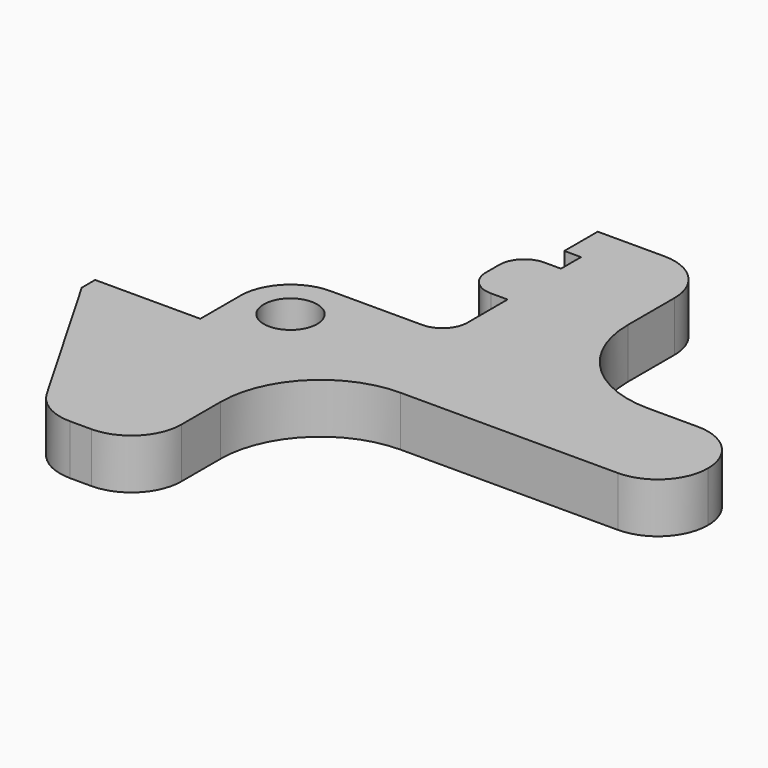
from build123d import *

# Parameters (mm, degrees)
F0_R     = 1.6
F0_W     = 6.3
F0_H     = 1
F0_W_2   = 2.5
F0_H_2   = 4
F1_DEPTH = 3
F2_R     = 2.99999
F3_R     = 6
F4_R     = 1.5


# Not quite as in the source:
# - a fillet or chamfer is up to 0.001 mm smaller than in the source, because OpenCascade refuses the exact size


with BuildPart() as f1:
    # F0 (on Top) → F1 (new body)
    with BuildSketch(Plane.XY):
        with BuildLine():
            ThreePointArc((0, 3), (-2.1213203436, 2.1213203436), (-3, 0))
            Line((-3, 0), (-3, -3))
            Line((-3, -3), (-3, -4))
            Line((-3, -4), (-9.3, -4))
            Line((-9.3, -4), (-3, -14.9119200877))
            Line((-3, -14.9119200877), (3, -14.9119200877))
            Line((3, -14.9119200877), (3, -3))
            Line((3, -3), (25, -3))
            Line((25, -3), (25, 3))
            Line((25, 3), (13, 3))
            Line((13, 3), (7, 3))
            Line((7, 3), (0, 3))
        make_face()
        Circle(F0_R, mode=Mode.SUBTRACT)
        with Locations((-6.15, -3.5)):
            Rectangle(F0_W, F0_H)
        Polygon((7, 7.5), (7, 3), (13, 3), (13, 13), (7, 13), (7, 11.5), align=None)
        with Locations((5.75, 9.5)):
            Rectangle(F0_W_2, F0_H_2)
        Polygon((7, 13), (13, 13), (13, 15.5), (6, 15.5), (6, 13), align=None)
    extrude(amount=F1_DEPTH)

    # F2 (radius 3 in the source; OpenCascade refuses exactly that, so slightly less here)
    f2_edges = [f1.edges().sort_by_distance(p)[0] for p in [
        (-3, -14.91192, 1.5),
        (3, -14.91192, 1.5),
        (25, -3, 1.5),
        (25, 3, 1.5),
        (13, 15.5, 1.5),
    ]]
    fillet(f2_edges, radius=F2_R)

    # F3
    f3_edges = [f1.edges().sort_by_distance(p)[0] for p in [
        (3, -3, 1.5),
        (13, 3, 1.5),
    ]]
    fillet(f3_edges, radius=F3_R)

    # F4
    f4_edges = [f1.edges().sort_by_distance(p)[0] for p in [
        (4.5, 11.5, 1.5),
        (4.5, 7.5, 1.5),
        (7, 3, 1.5),
    ]]
    fillet(f4_edges, radius=F4_R)


solid = f1.part
